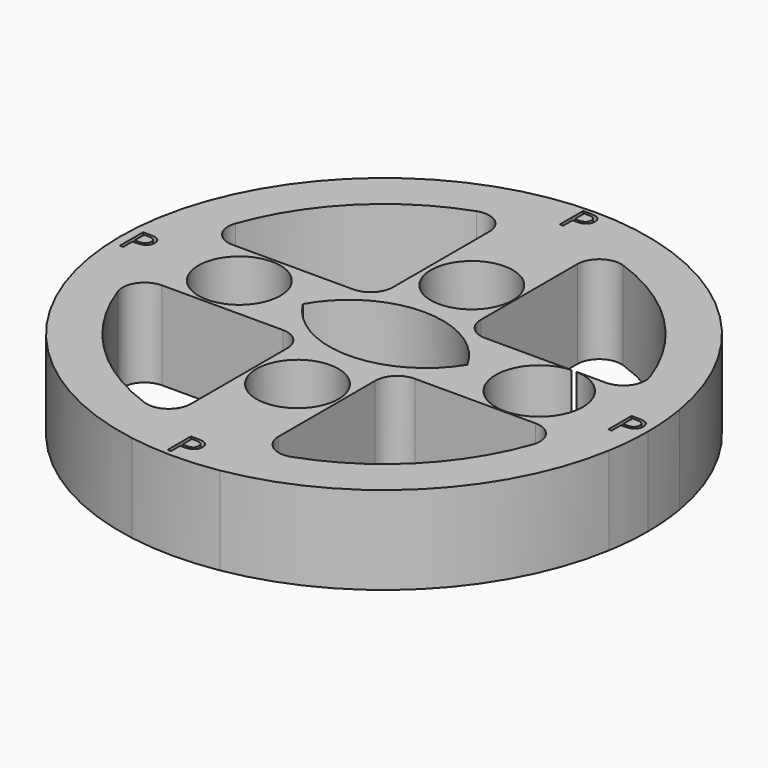
from build123d import *

# Parameters (mm, degrees)
F1_DEPTH     = 12.7
F2_R         = 11.835091
F3_DEPTH     = 77.47
F2_TEXT_SIZE = 11.772931
F4_DEPTH     = 87.884


# Not quite as in the source:
# - Text() gives the source's letters only with a copy of the font that has no kerning and outlines rounded to 1/6400 em; it was checked with that copy


with BuildPart() as f1:
    # F0 (on Top) → F1 (new body, symmetric)
    with BuildSketch(Plane.XY):
        with BuildLine():
            ThreePointArc((75.134213, -12.7), (75.933086, -6.372321), (76.2, 0))
            ThreePointArc((76.2, 0), (75.933086, 6.372321), (75.134213, 12.7))
            ThreePointArc((75.134213, 12.7), (53.881537, 53.881537), (12.7, 75.134213))
            ThreePointArc((12.7, 75.134213), (0, 76.2), (-12.7, 75.134213))
            ThreePointArc((-12.7, 75.134213), (-53.881537, 53.881537), (-75.134213, 12.7))
            ThreePointArc((-75.134213, 12.7), (-76.2, 0), (-75.134213, -12.7))
            ThreePointArc((-75.134213, -12.7), (-53.881537, -53.881537), (-12.7, -75.134213))
            ThreePointArc((-12.7, -75.134213), (0, -76.2), (12.7, -75.134213))
            ThreePointArc((12.7, -75.134213), (53.881537, -53.881537), (75.134213, -12.7))
        make_face()
        with BuildLine():
            ThreePointArc((-19.05, -12.7), (-14.559872, -14.559872), (-12.7, -19.05))
            Line((-12.7, -19.05), (-12.7, -53.881537))
            ThreePointArc((-12.7, -53.881537), (-15.383826, -59.06629), (-21.166667, -59.868374))
            ThreePointArc((-21.166667, -59.868374), (-44.901281, -44.901281), (-59.868374, -21.166667))
            ThreePointArc((-59.868374, -21.166667), (-59.06629, -15.383826), (-53.881537, -12.7))
            Line((-53.881537, -12.7), (-19.05, -12.7))
        make_face(mode=Mode.SUBTRACT)
        with BuildLine():
            Line((12.7, -53.881537), (12.7, -19.05))
            ThreePointArc((12.7, -19.05), (14.559872, -14.559872), (19.05, -12.7))
            Line((19.05, -12.7), (53.881537, -12.7))
            ThreePointArc((53.881537, -12.7), (59.06629, -15.383826), (59.868374, -21.166667))
            ThreePointArc((59.868374, -21.166667), (44.901281, -44.901281), (21.166667, -59.868374))
            ThreePointArc((21.166667, -59.868374), (15.383826, -59.06629), (12.7, -53.881537))
        make_face(mode=Mode.SUBTRACT)
        with BuildLine():
            ThreePointArc((-59.868374, 21.166667), (-44.901281, 44.901281), (-21.166667, 59.868374))
            ThreePointArc((-21.166667, 59.868374), (-15.383826, 59.06629), (-12.7, 53.881537))
            Line((-12.7, 53.881537), (-12.7, 19.05))
            ThreePointArc((-12.7, 19.05), (-14.559872, 14.559872), (-19.05, 12.7))
            Line((-19.05, 12.7), (-53.881537, 12.7))
            ThreePointArc((-53.881537, 12.7), (-59.06629, 15.383826), (-59.868374, 21.166667))
        make_face(mode=Mode.SUBTRACT)
        with BuildLine():
            ThreePointArc((0, 12.7), (8.980256, 8.980256), (12.7, 0))
            ThreePointArc((12.7, 0), (8.980256, -8.980256), (0, -12.7))
            ThreePointArc((0, -12.7), (-8.980256, -8.980256), (-12.7, 0))
            ThreePointArc((-12.7, 0), (-8.980256, 8.980256), (0, 12.7))
        make_face(mode=Mode.SUBTRACT)
        with BuildLine():
            ThreePointArc((19.05, 12.7), (14.559872, 14.559872), (12.7, 19.05))
            Line((12.7, 19.05), (12.7, 53.881537))
            ThreePointArc((12.7, 53.881537), (15.383826, 59.06629), (21.166667, 59.868374))
            ThreePointArc((21.166667, 59.868374), (44.901281, 44.901281), (59.868374, 21.166667))
            ThreePointArc((59.868374, 21.166667), (59.06629, 15.383826), (53.881537, 12.7))
            Line((53.881537, 12.7), (19.05, 12.7))
        make_face(mode=Mode.SUBTRACT)
    extrude(amount=F1_DEPTH, both=True)

    # F2 (on face) → F3 (cut)
    with BuildSketch(Plane.XY.offset(12.7)):
        with Locations((-41.762326, 0)):
            Circle(F2_R)
        with Locations((0, -31.218372)):
            Circle(F2_R)
        with BuildLine():
            ThreePointArc((-23.435674, 0), (0.310115, -13.178428), (24.055903, 0))
            ThreePointArc((24.055903, 0), (0.310115, 14.063747), (-23.435674, 0))
        make_face()
        with BuildLine():
            ThreePointArc((0, -12.7), (-8.980256, -8.980256), (-12.7, 0))
            ThreePointArc((-12.7, 0), (-8.980256, 8.980256), (0, 12.7))
            ThreePointArc((0, 12.7), (8.980256, 8.980256), (12.7, 0))
            ThreePointArc((12.7, 0), (8.980256, -8.980256), (0, -12.7))
        make_face(mode=Mode.SUBTRACT)
        with BuildLine():
            Line((43.9424, 12.7), (45.4656, 12.7))
            ThreePointArc((45.4656, 12.7), (44.704, 12.723094), (43.9424, 12.7))
        make_face()
        with BuildLine():
            ThreePointArc((43.9424, 12.7), (36.089485, -8.999714), (57.273514, 0.153581))
            ThreePointArc((57.273514, 0.153581), (53.857295, 8.768096), (45.4656, 12.7))
            Line((45.4656, 12.7), (43.9424, 12.7))
        make_face()
        with Locations((0.567068, 30.988)):
            Circle(F2_R)
    extrude(amount=-F3_DEPTH, mode=Mode.SUBTRACT)

    # F2 (on face) → F4 (cut)
    with BuildSketch(Plane.XY.offset(12.7)):
        with Locations((-74.611186, -3.519029)):
            Text('P', F2_TEXT_SIZE, font='Open Sans', text_align=(TextAlign.LEFT, TextAlign.BOTTOM))
        with Locations((67.398605, -4.755116)):
            Text('P', F2_TEXT_SIZE, font='Open Sans', text_align=(TextAlign.LEFT, TextAlign.BOTTOM))
        with Locations((-3.623855, 66.571627)):
            Text('P', F2_TEXT_SIZE, font='Open Sans', text_align=(TextAlign.LEFT, TextAlign.BOTTOM))
        with Locations((-3.928139, -74.634655)):
            Text('P', F2_TEXT_SIZE, font='Open Sans', text_align=(TextAlign.LEFT, TextAlign.BOTTOM))
    extrude(amount=-F4_DEPTH, mode=Mode.SUBTRACT)


solid = f1.part
